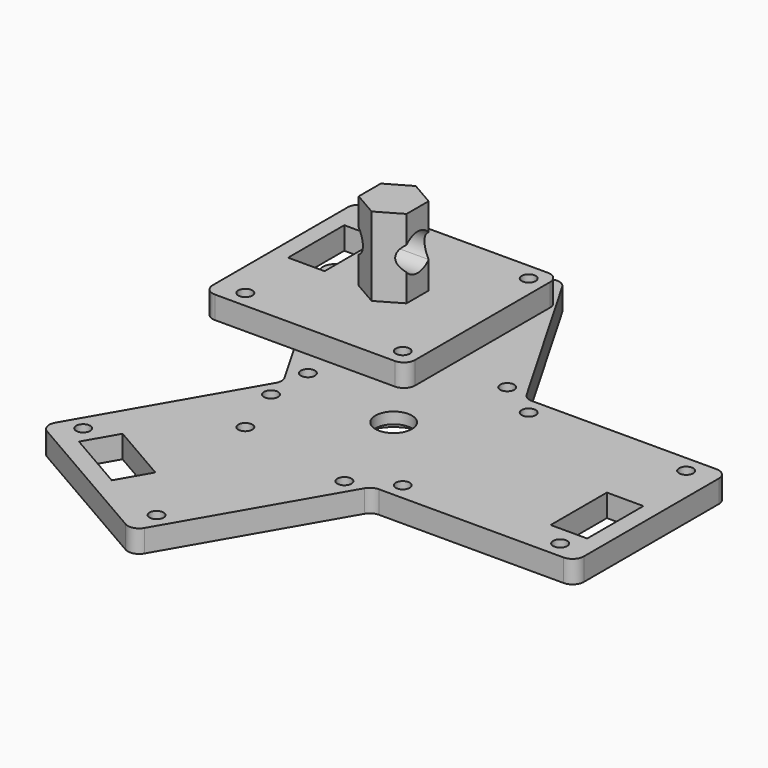
from build123d import *

# Parameters (mm, degrees)
F0_R           = 1.25
F0_W           = 36
F0_H           = 34
F0_W_2         = 6.5
F0_H_2         = 12.5
F0_R_2         = 6.25
F0_R_3         = 3.25
F1_DEPTH       = 4
F2_DEPTH       = 2
F3_R           = 2
F5_START       = 21
F4_W           = 36
F4_H           = 34
F4_R           = 1.25
F4_W_2         = 6.5
F4_H_2         = 12.5
F5_DEPTH       = 4
F6_D           = 2.5
F6_CBORE_D     = 5
F6_CBORE_DEPTH = 1.5
F8_DEPTH       = 14
F10_DEPTH      = 25
F11_R          = 2


with BuildPart() as f1:
    # F0 (on Top) → F1 (new body)
    with BuildSketch(Plane.XY):
        Polygon((-19.6299091524, 0), (9.8149545762, 17), (-8.1850454238, 48.1769145362), (-37.6299091524, 31.1769145362), align=None)
        with Locations((-18.5318329411, 4.0980762114)):
            Circle(F0_R, mode=Mode.SUBTRACT)
        with Locations((-32.5318329411, 28.3467875173)):
            Circle(F0_R, mode=Mode.SUBTRACT)
        Polygon((-9.0642105484, 36.6996732003), (-19.8895280957, 30.4496732003), (-23.1395280957, 36.0788383249), (-12.3142105484, 42.3288383249), align=None, mode=Mode.SUBTRACT)
        with Locations((-8.2831216351, 42.3467875173)):
            Circle(F0_R, mode=Mode.SUBTRACT)
        with Locations((5.7168783649, 18.0980762114)):
            Circle(F0_R, mode=Mode.SUBTRACT)
        with Locations((27.8149545762, 0)):
            Rectangle(F0_W, F0_H)
        with Locations((12.8149545762, -14)):
            Circle(F0_R, mode=Mode.SUBTRACT)
        with Locations((40.8149545762, -14)):
            Circle(F0_R, mode=Mode.SUBTRACT)
        with Locations((39.5649545762, -4.25)):
            Rectangle(F0_W_2, F0_H_2, mode=Mode.SUBTRACT)
        with Locations((12.8149545762, 14)):
            Circle(F0_R, mode=Mode.SUBTRACT)
        with Locations((40.8149545762, 14)):
            Circle(F0_R, mode=Mode.SUBTRACT)
        Polygon((-8.1850454238, -48.1769145362), (9.8149545762, -17), (-19.6299091524, 0), (-37.6299091524, -31.1769145362), align=None)
        with Locations((-32.5318329411, -28.3467875173)):
            Circle(F0_R, mode=Mode.SUBTRACT)
        Polygon((-27.2507440278, -26.1996732003), (-16.4254264805, -32.4496732003), (-19.6754264805, -38.0788383249), (-30.5007440278, -31.8288383249), align=None, mode=Mode.SUBTRACT)
        with Locations((-8.2831216351, -42.3467875173)):
            Circle(F0_R, mode=Mode.SUBTRACT)
        with Locations((-18.5318329411, -4.0980762114)):
            Circle(F0_R, mode=Mode.SUBTRACT)
        with Locations((5.7168783649, -18.0980762114)):
            Circle(F0_R, mode=Mode.SUBTRACT)
        Polygon((9.8149545762, -17), (9.8149545762, 17), (-19.6299091524, 0), align=None)
        Circle(F0_R_2, mode=Mode.SUBTRACT)
        Circle(F0_R_2)
        Circle(F0_R_3, mode=Mode.SUBTRACT)
    extrude(amount=F1_DEPTH)

    # F0 (on Top) → F2 (cut)
    with BuildSketch(Plane.XY):
        Circle(F0_R_2)
        Circle(F0_R_3, mode=Mode.SUBTRACT)
    extrude(amount=F2_DEPTH, mode=Mode.SUBTRACT)

    # F3
    f3_edges = [f1.edges().sort_by_distance(p)[0] for p in [
        (-8.185045, 48.176915, 2),
        (45.814955, 17, 2),
        (45.814955, -17, 2),
        (9.814955, -17, 2),
        (-8.185045, -48.176915, 2),
        (-37.629909, -31.176915, 2),
        (-19.629909, 0, 2),
        (-37.629909, 31.176915, 2),
        (9.814955, 17, 2),
    ]]
    fillet(f3_edges, radius=F3_R)

    # F6 (through all)
    with Locations(Plane(origin=(0, 0, 0), x_dir=(1, 0, 0), z_dir=(0, 0, -1))):
        with Locations((-15.1850454238, -14), (-15.1850454238, 14)):
            CounterBoreHole(F6_D / 2, F6_CBORE_D / 2, F6_CBORE_DEPTH)


with BuildPart() as f5:
    # F4 (on Top) → F5 (new body)
    with BuildSketch(Plane.XY.offset(F5_START)):
        with Locations((-2.1850454238, 0)):
            Rectangle(F4_W, F4_H)
        with Locations((-15.1850454238, -14)):
            Circle(F4_R, mode=Mode.SUBTRACT)
        with Locations((12.8149545762, -14)):
            Circle(F4_R, mode=Mode.SUBTRACT)
        with Locations((-13.9350454238, 4.25)):
            Rectangle(F4_W_2, F4_H_2, mode=Mode.SUBTRACT)
        with Locations((-15.1850454238, 14)):
            Circle(F4_R, mode=Mode.SUBTRACT)
        with Locations((12.8149545762, 14)):
            Circle(F4_R, mode=Mode.SUBTRACT)
    extrude(amount=F5_DEPTH)

    # F7 (on face) → F8 (join)
    with BuildSketch(Plane.XY.offset(25)):
        Polygon((4.25, -2.4537386441), (4.25, 2.4537386441), (0, 4.9074772881), (-4.25, 2.4537386441), (-4.25, -2.4537386441), (0, -4.9074772881), align=None)
    extrude(amount=F8_DEPTH)

    # F9 (on face) → F10 (cut)
    with BuildSketch(Plane(origin=(-4.25, 0, 0), x_dir=(0, -1, 0), z_dir=(-1, 0, 0))):
        with BuildLine():
            Line((2.4537386441, 29.8688813579), (2.4537386441, 34.1311186421))
            ThreePointArc((2.4537386441, 34.1311186421), (0, 35.25), (-2.4537386441, 34.1311186421))
            Line((-2.4537386441, 34.1311186421), (-2.4537386441, 29.8688813579))
            ThreePointArc((-2.4537386441, 29.8688813579), (0, 28.75), (2.4537386441, 29.8688813579))
        make_face()
        with BuildLine():
            Line((-2.4537386441, 29.8688813579), (-2.4537386441, 34.1311186421))
            ThreePointArc((-2.4537386441, 34.1311186421), (-3.25, 32), (-2.4537386441, 29.8688813579))
        make_face()
        with BuildLine():
            ThreePointArc((2.4537386441, 29.8688813579), (3.0444334935, 30.8624918886), (3.25, 32))
            ThreePointArc((3.25, 32), (3.0444334935, 33.1375081114), (2.4537386441, 34.1311186421))
            Line((2.4537386441, 34.1311186421), (2.4537386441, 29.8688813579))
        make_face()
    extrude(amount=-F10_DEPTH, mode=Mode.SUBTRACT)

    # F11
    f11_edges = [f5.edges().sort_by_distance(p)[0] for p in [
        (15.814955, -17, 23),
        (15.814955, 17, 23),
        (-20.185045, 17, 23),
        (-20.185045, -17, 23),
    ]]
    fillet(f11_edges, radius=F11_R)


solid = Compound([f1.part, f5.part])
